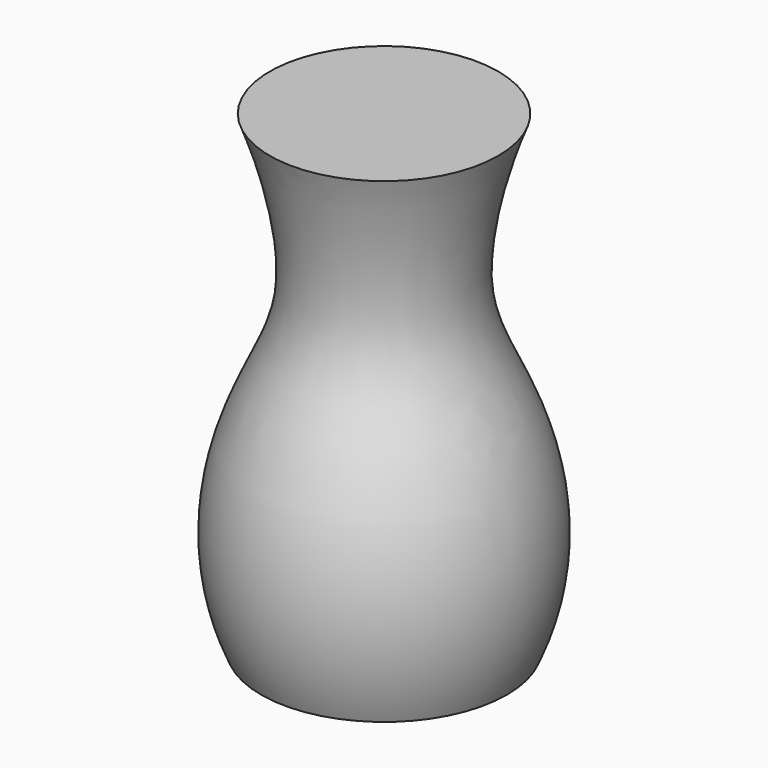
from build123d import *


with BuildPart() as f1:
    # F0 (on Front) → F1 (revolve)
    with BuildSketch(Plane.XZ):
        with BuildLine():
            Line((0, 115), (0, 0))
            Line((0, 0), (30, 0))
            add(Edge.make_bspline(
                [(30, 0), (38.8833321077, 19.9206599167), (32.5653867482, 52.190924217), (16.0278789821, 75.5819524262), (23.8774344325, 104.9342304468), (27.8661828488, 115)],
                knots=[0, 0, 0, 0, 0.3862215976, 0.6683274414, 1, 1, 1, 1], degree=3))
            Line((27.8661828488, 115), (0, 115))
        make_face()
    revolve(axis=Axis((0, 0, 57.5), (0, 0, 1)))


solid = f1.part
